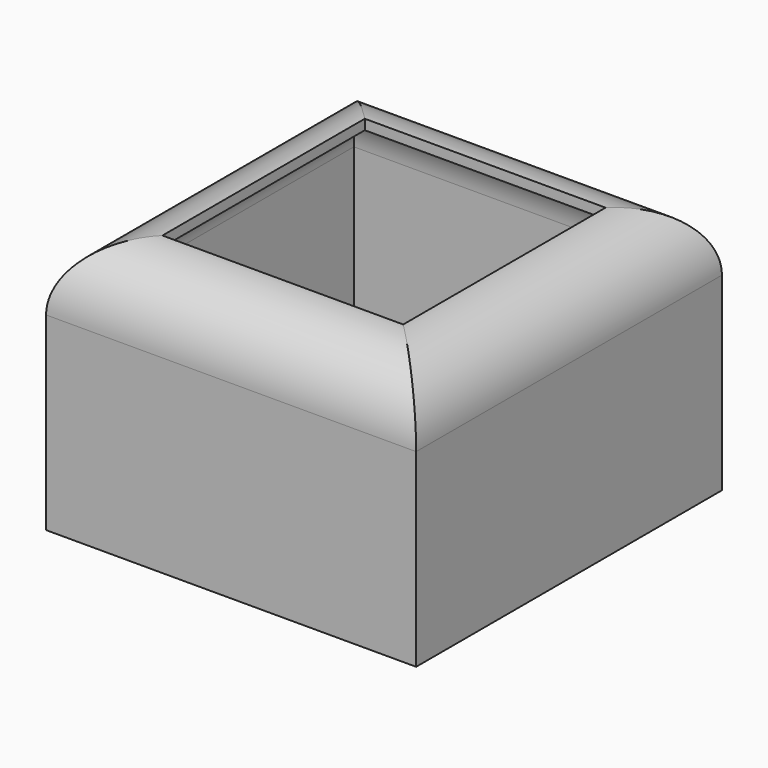
from build123d import *

# Parameters (mm, degrees)
F0_W     = 92.8067304194
F0_H     = 95.8546847105
F1_DEPTH = 63.7208949775
F2_R     = 16.2105709048
F3_T     = -2.54


# Not quite as in the source:
# - a shell that OpenCascade refuses in one call is made with other operations: the cavity is built on its own and cut out


with BuildPart() as f1:
    # F0 (on Top) → F1 (new body)
    with BuildSketch(Plane.XY):
        with Locations((0.6604772061, -2.7937293053)):
            Rectangle(F0_W, F0_H)
    extrude(amount=F1_DEPTH)

    # F2
    f2_edges = [f1.edges().sort_by_distance(p)[0] for p in [
        (-45.742888, -2.793729, 63.720895),
        (0.660477, -50.721072, 63.720895),
        (47.063842, -2.793729, 63.720895),
        (0.660477, 45.133613, 63.720895),
    ]]
    fillet(f2_edges, radius=F2_R)

    # F3: a shell. OpenCascade refuses it in one call, so the cavity is built on its own and cut out:
    # the body offset inwards by the wall thickness, plus a prism from it out through each open face.
    f3_core = offset(f1.part, amount=F3_T, mode=Mode.PRIVATE)
    f3_exits = [f3_core.faces().sort_by_distance(p)[0] for p in [
        (0.660477, -2.793729, 61.180895),
    ]]
    add(f3_core, mode=Mode.SUBTRACT)
    extrude(f3_exits, amount=-F3_T, mode=Mode.SUBTRACT)


solid = f1.part
